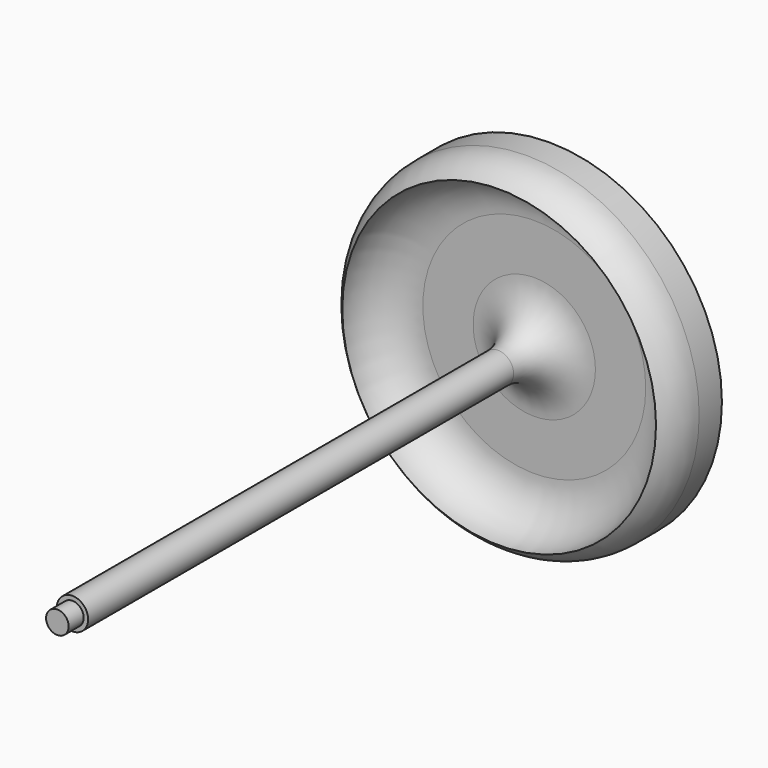
from build123d import *

# Parameters (mm, degrees)
F0_R     = 31.75
F0_R_2   = 3.175
F1_DEPTH = 3.81
F2_DEPTH = 124.46
F0_R_3   = 34.925
F3_DEPTH = 12.7
F5_R     = 3.175
F5_R_2   = 2.286
F6_DEPTH = 3.81


# Not quite as in the source:
# - a fillet or chamfer that OpenCascade refuses, or shapes differently, is made with other operations: its cross-section is extruded or revolved along the edge and cut away or added


with BuildPart() as f1:
    # F0 (on Front) → F1 (new body)
    with BuildSketch(Plane.XZ):
        Circle(F0_R)
        Circle(F0_R_2, mode=Mode.SUBTRACT)
        Circle(F0_R_2)
    extrude(amount=F1_DEPTH)

    # F0 (on Front) → F2 (join)
    with BuildSketch(Plane.XZ):
        Circle(F0_R_2)
    extrude(amount=F2_DEPTH)

    # F0 (on Front) → F3 (join)
    with BuildSketch(Plane.XZ):
        Circle(F0_R_3)
        Circle(F0_R, mode=Mode.SUBTRACT)
    extrude(amount=F3_DEPTH)

    # F4: fillet of radius 9.1981536726 on 3 edges, made by hand

    # F4_s1 → F4_t2 (revolve)
    with BuildSketch(Plane.XY):
        with BuildLine():
            ThreePointArc((31.75, -12.7), (28.9512095664, -6.3960255802), (22.5570096106, -3.81))
            Line((22.5570096106, -3.81), (31.75, -3.81))
            Line((31.75, -3.81), (31.75, -12.7))
        make_face()
    revolve(axis=Axis((0, -3.81, 0), (0, -1, 0)))

    # F4_s3 → F4_t4 (revolve)
    with BuildSketch(Plane.XY):
        with BuildLine():
            ThreePointArc((12.3731536726, -3.81), (5.8690768363, -6.5040768363), (3.175, -13.0081536726))
            Line((3.175, -13.0081536726), (3.175, -3.81))
            Line((3.175, -3.81), (12.3731536726, -3.81))
        make_face()
    revolve(axis=Axis((0, -3.81, 0), (0, 1, 0)))

    # F4_s5 → F4_t6 (revolve, cut)
    with BuildSketch(Plane.XY):
        with BuildLine():
            ThreePointArc((34.925, -5.7481908239), (34.0936833659, -9.5694561844), (31.75, -12.7))
            Line((31.75, -12.7), (34.925, -12.7))
            Line((34.925, -12.7), (34.925, -5.7481908239))
        make_face()
    revolve(axis=Axis((0, -12.7, 0), (0, -1, 0)), mode=Mode.SUBTRACT)

    # F5 (on face) → F6 (cut)
    with BuildSketch(Plane.XZ.offset(124.46)):
        Circle(F5_R)
        Circle(F5_R_2, mode=Mode.SUBTRACT)
    extrude(amount=-F6_DEPTH, mode=Mode.SUBTRACT)


solid = f1.part
